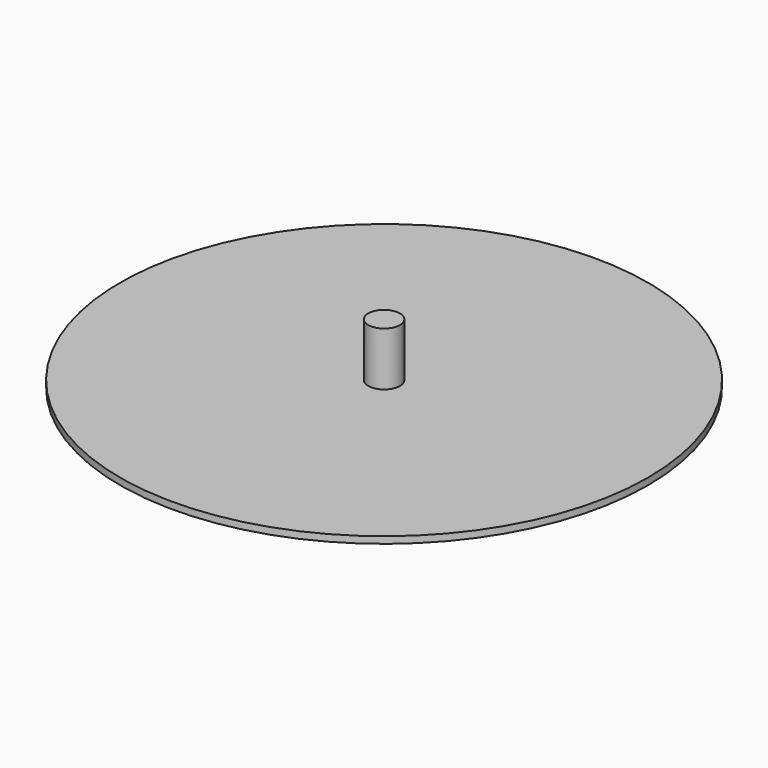
from build123d import *

# Parameters (mm, degrees)
F0_R     = 125
F0_R_2   = 63.5
F1_DEPTH = 3.2
F2_R     = 7.5
F3_DEPTH = 25.4


with BuildPart() as f1:
    # F0 (on Top) → F1 (new body)
    with BuildSketch(Plane.XY):
        Circle(F0_R)
        Circle(F0_R_2, mode=Mode.SUBTRACT)
        Circle(F0_R_2)
    extrude(amount=F1_DEPTH)

    # F2 (on face) → F3 (join)
    with BuildSketch(Plane.XY.offset(3.2)):
        Circle(F2_R)
    extrude(amount=F3_DEPTH)


solid = f1.part
